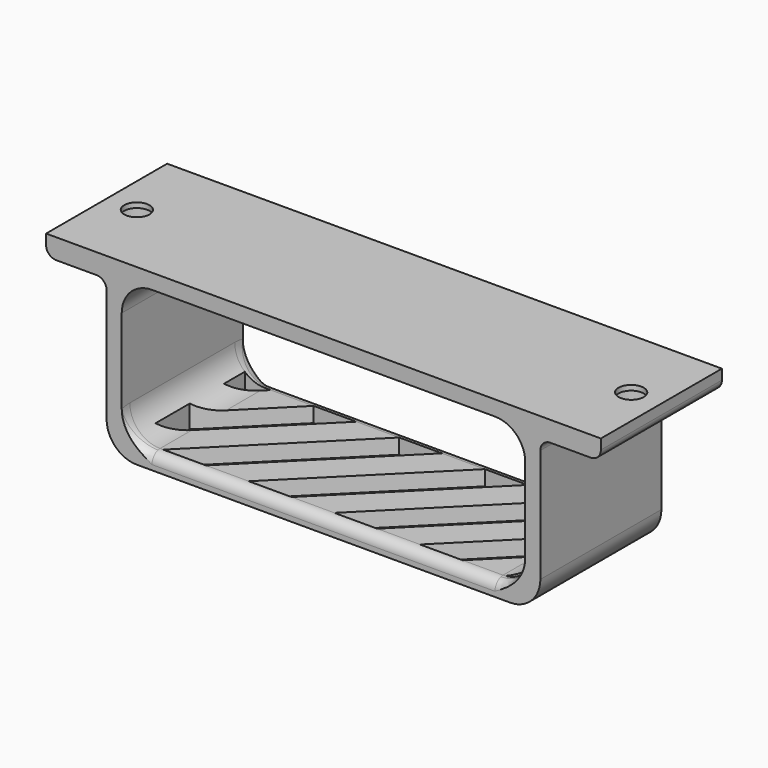
from build123d import *

# Parameters (mm, degrees)
F0_W     = 80
F0_H     = 28.5
F0_W_2   = 12
F0_H_2   = 4
F2_DEPTH = 30
F3_R     = 2
F4_R     = 2.5
F5_DEPTH = 17.25
F6_R     = 6
F8_DEPTH = 17.25
F4_R_2   = 4.125
F9_DEPTH = 16.25


# Not quite as in the source:
# - two fillets or chamfers of one size are made in one step


with BuildPart() as f2:
    # F0 (on Front) → F2 (new body)
    with BuildSketch(Plane.XZ):
        Polygon((43, 17.25), (-43, 17.25), (-43, 13.25), (-43, -17.25), (43, -17.25), (43, 13.25), align=None)
        Rectangle(F0_W, F0_H, mode=Mode.SUBTRACT)
        with Locations((49, 15.25)):
            Rectangle(F0_W_2, F0_H_2)
        with Locations((-49, 15.25)):
            Rectangle(F0_W_2, F0_H_2)
    extrude(amount=-F2_DEPTH)

    # F3
    f3_edges = [f2.edges().sort_by_distance(p)[0] for p in [
        (0, 0, -14.25),
        (0, 30, -14.25),
        (-43, 15, 13.25),
        (43, 15, 13.25),
        (55, 15, 13.25),
        (-55, 15, 13.25),
    ]]
    fillet(f3_edges, radius=F3_R)

    # F4 (on Top) → F5 (cut, through all)
    with BuildSketch(Plane.XY):
        with Locations((49, 15)):
            Circle(F4_R)
        with Locations((-49, 15)):
            Circle(F4_R)
    extrude(amount=F5_DEPTH, mode=Mode.SUBTRACT)

    # F6 (call 1 of 6: OpenCascade refuses the feature's edges together)
    f6_edges = [f2.edges().sort_by_distance(p)[0] for p in [
        (-40, 15, 14.25),
    ]]
    fillet(f6_edges, radius=F6_R)

    # F6#2 (call 2 of 6)
    f6_2_edges = [f2.edges().sort_by_distance(p)[0] for p in [
        (-40, 15, -14.25),
    ]]
    fillet(f6_2_edges, radius=F6_R)

    # F6#3 (call 3 of 6)
    f6_3_edges = [f2.edges().sort_by_distance(p)[0] for p in [
        (40, 15, 14.25),
    ]]
    fillet(f6_3_edges, radius=F6_R)

    # F6#4 (call 4 of 6)
    f6_4_edges = [f2.edges().sort_by_distance(p)[0] for p in [
        (40, 15, -14.25),
    ]]
    fillet(f6_4_edges, radius=F6_R)

    # F6#5 (call 5 of 6)
    f6_5_edges = [f2.edges().sort_by_distance(p)[0] for p in [
        (-43, 15, -17.25),
    ]]
    fillet(f6_5_edges, radius=F6_R)

    # F6#6 (call 6 of 6)
    f6_6_edges = [f2.edges().sort_by_distance(p)[0] for p in [
        (43, 15, -17.25),
    ]]
    fillet(f6_6_edges, radius=F6_R)

    # F1 (on Top) → F8 (cut, through all)
    with BuildSketch(Plane.XY):
        Polygon((38, 2), (38, 5.5), (34.5, 2), align=None)
        Polygon((38, 13.9852813742), (38, 22.4705627485), (17.5294372515, 2), (26.0147186258, 2), align=None)
        Polygon((9.0441558773, 2), (35.0441558773, 28), (26.558874503, 28), (0.558874503, 2), align=None)
        Polygon((-7.9264068712, 2), (18.0735931288, 28), (9.5883117546, 28), (-16.4116882454, 2), align=None)
        Polygon((-24.8969696197, 2), (1.1030303803, 28), (-7.3822509939, 28), (-33.3822509939, 2), align=None)
        Polygon((-38, 5.8675323681), (-15.8675323681, 28), (-24.3528137424, 28), (-38, 14.3528137424), align=None)
        Polygon((-38, 22.8380951166), (-32.8380951166, 28), (-38, 28), align=None)
    extrude(amount=-F8_DEPTH, mode=Mode.SUBTRACT)

    # F4 (on Top) → F9 (cut)
    with BuildSketch(Plane.XY):
        with Locations((-49, 15)):
            Circle(F4_R_2)
        with Locations((-49, 15)):
            Circle(F4_R, mode=Mode.SUBTRACT)
        with Locations((49, 15)):
            Circle(F4_R_2)
        with Locations((49, 15)):
            Circle(F4_R, mode=Mode.SUBTRACT)
    extrude(amount=F9_DEPTH, mode=Mode.SUBTRACT)


solid = f2.part
